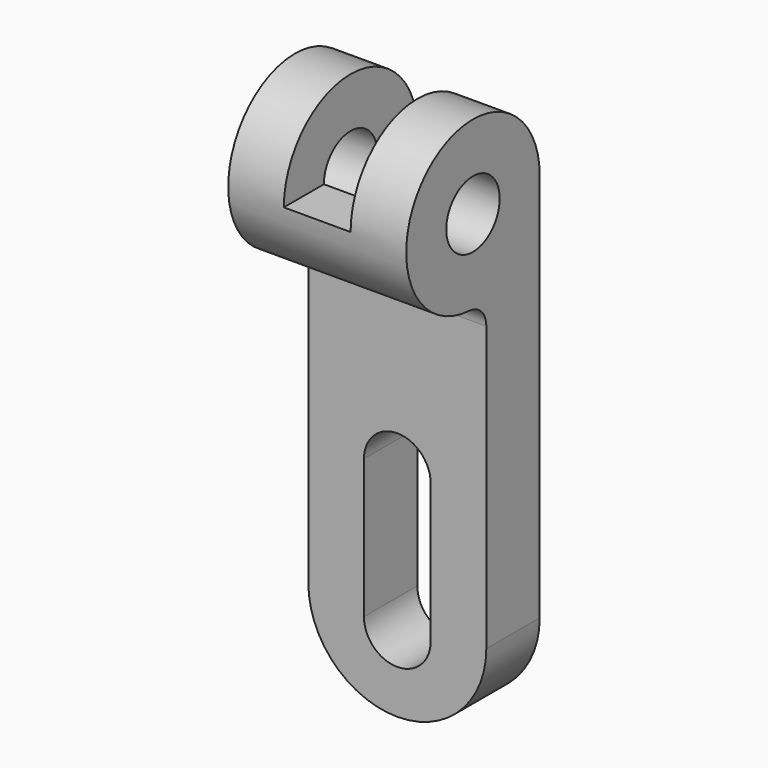
from build123d import *

# Parameters (mm, degrees)
F0_R     = 6
F1_DEPTH = 32
F3_DEPTH = 15.001
F4_W     = 12
F4_H     = 15
F5_DEPTH = 30.001


# Not quite as in the source:
# - a feature names something its author has since deleted; it is built from what else it names


with BuildPart() as f1:
    # F0 (on Right) → F1 (new body)
    with BuildSketch(Plane.YZ):
        with BuildLine():
            Line((15, -86), (15, 0))
            ThreePointArc((15, 0), (-10.3237080242, 10.8821437517), (-0.7894736842, -14.9792099692))
            ThreePointArc((-0.7894736842, -14.9792099692), (1.9019050004, -16.2206771546), (3, -18.973665961))
            Line((3, -18.973665961), (3, -86))
            Line((3, -86), (15, -86))
        make_face()
        Circle(F0_R, mode=Mode.SUBTRACT)
    extrude(amount=-F1_DEPTH)

    # F2 (on Front) → F3 (cut, through all)
    with BuildSketch(Plane.XZ):
        with BuildLine():
            ThreePointArc((-16, -86), (-27.313708499, -81.313708499), (-32, -70))
            Line((-32, -70), (-32, -86))
            Line((-32, -86), (-16, -86))
        make_face()
        with BuildLine():
            ThreePointArc((0, -70), (-4.686291501, -81.313708499), (-16, -86))
            Line((-16, -86), (0, -86))
            Line((0, -86), (0, -70))
        make_face()
        with BuildLine():
            Line((-10, -72.1075447824), (-10, -47.1075447824))
            ThreePointArc((-10, -47.1075447824), (-16, -41.1075447824), (-22, -47.1075447824))
            Line((-22, -47.1075447824), (-22, -72.1075447824))
            ThreePointArc((-22, -72.1075447824), (-16, -78.1075447824), (-10, -72.1075447824))
        make_face()
    extrude(amount=-F3_DEPTH, mode=Mode.SUBTRACT)

    # F4 (on face) → F5 (cut, through all)
    with BuildSketch(Plane(origin=(0, 15, 0), x_dir=(-1, 0, 0), z_dir=(0, 1, 0))):
        with Locations((16, 7.5)):
            Rectangle(F4_W, F4_H)
    extrude(amount=-F5_DEPTH, mode=Mode.SUBTRACT)


solid = f1.part
